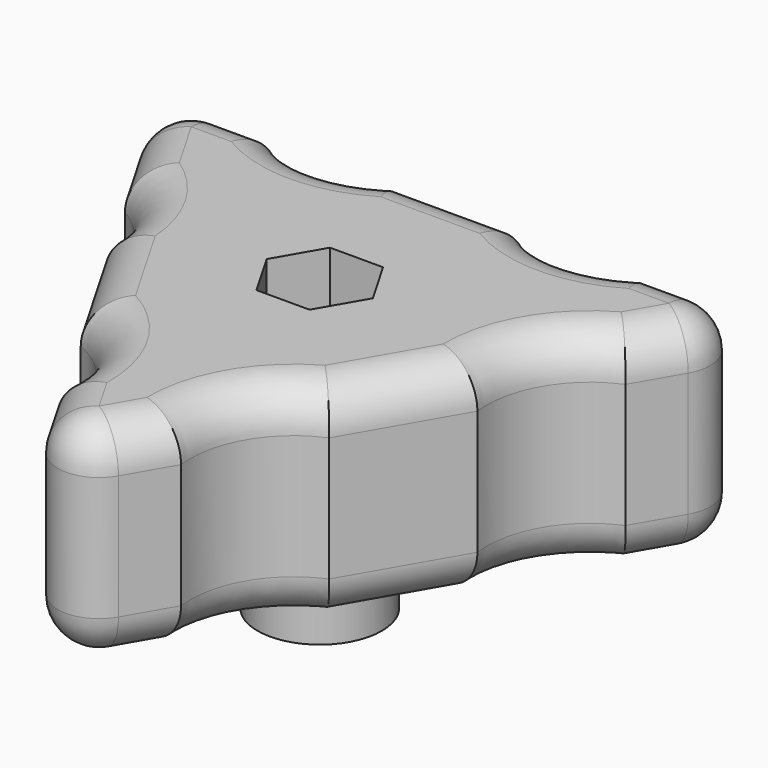
from build123d import *

# Parameters (mm, degrees)
F1_DEPTH     = 25.4
F2_R         = 5.08
F3_R         = 5.08
F4_T1_DEPTH  = 15.24
F4_T6_DEPTH  = 5.08
F4_T12_DEPTH = 5.08
F4_T18_DEPTH = 5.08
F4_T24_DEPTH = 5.08
F4_T30_DEPTH = 5.08
F4_T36_DEPTH = 5.08
F5_R         = 7.62
F6_DEPTH     = 10.16
F8_DEPTH     = 38.1


# Not quite as in the source:
# - a fillet or chamfer that OpenCascade refuses, or shapes differently, is made with other operations: its cross-section is extruded or revolved along the edge and cut away or added


with BuildPart() as f1:
    # F0 (on Top) → F1 (new body)
    with BuildSketch(Plane.XY):
        with BuildLine():
            Line((-22.8599986406, 21.9970466689), (-38.0999986406, 21.9970476107))
            Line((-38.0999986406, 21.9970476107), (-29.3011817939, 6.7570476107))
            ThreePointArc((-29.3011817939, 6.7570476107), (-24.5610386949, 2.0561338123), (-22.8600002719, -4.3994076385))
            Line((-22.8600002719, -4.3994076385), (-15.2400010875, -17.5976352631))
            ThreePointArc((-15.2400010875, -17.5976352631), (-9.2302968913, -22.9267492113), (-7.6200019032, -30.7958628877))
            Line((-7.6200019032, -30.7958628877), (-2.7189e-06, -43.9940905122))
            Line((-2.7189e-06, -43.9940905122), (7.6199980968, -30.7958638295))
            ThreePointArc((7.6199980968, -30.7958638295), (9.2302940575, -22.9267503522), (15.2399989124, -17.5976371467))
            Line((15.2399989124, -17.5976371467), (22.8599997281, -4.399410464))
            ThreePointArc((22.8599997281, -4.399410464), (24.4702956888, 3.4697030133), (30.4800005438, 8.7988162188))
            Line((30.4800005438, 8.7988162188), (38.1000013594, 21.9970429015))
            Line((38.1000013594, 21.9970429015), (22.8600013594, 21.9970438434))
            ThreePointArc((22.8600013594, 21.9970438434), (15.2400012025, 19.4570443143), (7.6200013594, 21.9970447852))
            Line((7.6200013594, 21.9970447852), (-7.6199986406, 21.997045727))
            ThreePointArc((-7.6199986406, 21.997045727), (-15.2399987975, 19.457046198), (-22.8599986406, 21.9970466689))
        make_face()
    extrude(amount=F1_DEPTH)

    # F2
    f2_edges = [f1.edges().sort_by_distance(p)[0] for p in [
        (-30.479999, 21.997047, 25.4),
        (-33.70059, 14.377048, 25.4),
        (-24.561039, 2.056134, 25.4),
        (-19.050001, -10.998521, 25.4),
        (-9.230297, -22.926749, 25.4),
        (-3.810002, -37.394977, 25.4),
        (3.809998, -37.394977, 25.4),
        (9.230294, -22.92675, 25.4),
        (19.049999, -10.998524, 25.4),
        (24.470296, 3.469703, 25.4),
        (34.290001, 15.39793, 25.4),
        (30.480001, 21.997043, 25.4),
        (15.240001, 19.457044, 25.4),
        (1e-06, 21.997045, 25.4),
        (-15.239999, 19.457046, 25.4),
    ]]
    fillet(f2_edges, radius=F2_R)

    # F3
    f3_edges = [f1.edges().sort_by_distance(p)[0] for p in [
        (-30.479999, 21.997047, 0),
        (-33.70059, 14.377048, 0),
        (-24.561039, 2.056134, 0),
        (-19.050001, -10.998521, 0),
        (-9.230297, -22.926749, 0),
        (-3.810002, -37.394977, 0),
        (3.809998, -37.394977, 0),
        (9.230294, -22.92675, 0),
        (19.049999, -10.998524, 0),
        (24.470296, 3.469703, 0),
        (34.290001, 15.39793, 0),
        (30.480001, 21.997043, 0),
        (15.240001, 19.457044, 0),
        (1e-06, 21.997045, 0),
        (-15.239999, 19.457046, 0),
    ]]
    fillet(f3_edges, radius=F3_R)

    # F4: fillet of radius 5.08 on 3 edges, made by hand

    # F4_s2 → F4_t1 (cut)
    with BuildSketch(Plane.XY.offset(5.08)):
        with BuildLine():
            ThreePointArc((-4.3994112992, -36.3740902404), (-2.4049e-06, -38.9140905122), (4.3994068033, -36.3740907841))
            Line((4.3994068033, -36.3740907841), (-2.7189e-06, -43.9940905122))
            Line((-2.7189e-06, -43.9940905122), (-4.3994112992, -36.3740902404))
        make_face()
        with BuildLine():
            ThreePointArc((29.301183257, 21.9970434453), (33.7005921512, 19.4570431734), (33.7005918373, 14.3770431734))
            Line((33.7005918373, 14.3770431734), (38.1000013594, 21.9970429015))
            Line((38.1000013594, 21.9970429015), (29.301183257, 21.9970434453))
        make_face()
        with BuildLine():
            ThreePointArc((-29.3011805381, 21.997047067), (-33.7005897463, 19.4570473389), (-33.7005900603, 14.3770473389))
            Line((-33.7005900603, 14.3770473389), (-38.0999986406, 21.9970476107))
            Line((-38.0999986406, 21.9970476107), (-29.3011805381, 21.997047067))
        make_face()
    extrude(amount=F4_T1_DEPTH, mode=Mode.SUBTRACT)


with BuildPart() as f4_tool4:
    # F4_s5 → F4_t6 (new body)
    with BuildSketch(Plane.XY.offset(20.32)):
        Polygon((-29.3011808521, 16.917047067), (-29.3011805381, 21.997047067), (-38.0999986406, 21.9970476107), (-33.7005900603, 14.3770473389), align=None)
    extrude(amount=F4_T6_DEPTH)

    # F4_s7 → F4_t8 (revolve, cut)
    with BuildSketch(Plane(origin=(-29.3011808521, 16.917047067, 20.32), x_dir=(0.8660253729, -0.5000000535, 0), z_dir=(-0.5000000535, -0.8660253729, 0))):
        with BuildLine():
            ThreePointArc((0, -5.08), (5.08, 0), (0, 5.08))
            Line((0, 5.08), (0, -5.08))
        make_face()
    revolve(axis=Axis((-29.3011808521, 16.917047067, 20.32), (0, 0, 1)), mode=Mode.SUBTRACT)


with BuildPart() as f1_1:
    add(f1.part)

    # F4_t3: cut F4_tool4
    add(f4_tool4.part, mode=Mode.SUBTRACT)


with BuildPart() as f4_tool10:
    # F4_s11 → F4_t12 (new body)
    with BuildSketch(Plane.XY.offset(20.32)):
        Polygon((29.301182943, 16.9170434453), (29.301183257, 21.9970434453), (38.1000013594, 21.9970429015), (33.7005918373, 14.3770431734), align=None)
    extrude(amount=F4_T12_DEPTH)

    # F4_s13 → F4_t14 (revolve, cut)
    with BuildSketch(Plane(origin=(29.301182943, 16.9170434453, 20.32), x_dir=(-0.8660254347, -0.4999999465, 0), z_dir=(-0.4999999465, 0.8660254347, 0))):
        with BuildLine():
            ThreePointArc((0, -5.08), (5.08, 0), (0, 5.08))
            Line((0, 5.08), (0, -5.08))
        make_face()
    revolve(axis=Axis((29.301182943, 16.9170434453, 20.32), (0, 0, 1)), mode=Mode.SUBTRACT)


with BuildPart() as f1_2:
    add(f1_1.part)

    # F4_t9: cut F4_tool10
    add(f4_tool10.part, mode=Mode.SUBTRACT)


with BuildPart() as f4_tool16:
    # F4_s17 → F4_t18 (new body)
    with BuildSketch(Plane.XY.offset(5.08)):
        Polygon((-2.091e-06, -33.8340905122), (-4.3994112992, -36.3740902404), (-2.7189e-06, -43.9940905122), (4.3994068033, -36.3740907841), align=None)
    extrude(amount=-F4_T18_DEPTH)

    # F4_s19 → F4_t20 (revolve, cut)
    with BuildSketch(Plane(origin=(-2.091e-06, -33.8340905122, 5.08), x_dir=(6.18e-08, 1, 0), z_dir=(-1, 6.18e-08, 0))):
        with BuildLine():
            ThreePointArc((0, -5.08), (5.08, 0), (0, 5.08))
            Line((0, 5.08), (0, -5.08))
        make_face()
    revolve(axis=Axis((-2.091e-06, -33.8340905122, 5.08), (0, 0, -1)), mode=Mode.SUBTRACT)


with BuildPart() as f1_3:
    add(f1_2.part)

    # F4_t15: cut F4_tool16
    add(f4_tool16.part, mode=Mode.SUBTRACT)


with BuildPart() as f4_tool22:
    # F4_s23 → F4_t24 (new body)
    with BuildSketch(Plane.XY.offset(20.32)):
        Polygon((-2.091e-06, -33.8340905122), (-4.3994112992, -36.3740902404), (-2.7189e-06, -43.9940905122), (4.3994068033, -36.3740907841), align=None)
    extrude(amount=F4_T24_DEPTH)

    # F4_s25 → F4_t26 (revolve, cut)
    with BuildSketch(Plane(origin=(-2.091e-06, -33.8340905122, 20.32), x_dir=(6.18e-08, 1, 0), z_dir=(1, -6.18e-08, 0))):
        with BuildLine():
            ThreePointArc((0, -5.08), (5.08, 0), (0, 5.08))
            Line((0, 5.08), (0, -5.08))
        make_face()
    revolve(axis=Axis((-2.091e-06, -33.8340905122, 20.32), (0, 0, 1)), mode=Mode.SUBTRACT)


with BuildPart() as f1_4:
    add(f1_3.part)

    # F4_t21: cut F4_tool22
    add(f4_tool22.part, mode=Mode.SUBTRACT)


with BuildPart() as f4_tool28:
    # F4_s29 → F4_t30 (new body)
    with BuildSketch(Plane.XY.offset(5.08)):
        Polygon((29.301182943, 16.9170434453), (29.301183257, 21.9970434453), (38.1000013594, 21.9970429015), (33.7005918373, 14.3770431734), align=None)
    extrude(amount=-F4_T30_DEPTH)

    # F4_s31 → F4_t32 (revolve, cut)
    with BuildSketch(Plane(origin=(29.301182943, 16.9170434453, 5.08), x_dir=(-0.8660254347, -0.4999999465, 0), z_dir=(0.4999999465, -0.8660254347, 0))):
        with BuildLine():
            ThreePointArc((0, -5.08), (5.08, 0), (0, 5.08))
            Line((0, 5.08), (0, -5.08))
        make_face()
    revolve(axis=Axis((29.301182943, 16.9170434453, 5.08), (0, 0, -1)), mode=Mode.SUBTRACT)


with BuildPart() as f1_5:
    add(f1_4.part)

    # F4_t27: cut F4_tool28
    add(f4_tool28.part, mode=Mode.SUBTRACT)


with BuildPart() as f4_tool34:
    # F4_s35 → F4_t36 (new body)
    with BuildSketch(Plane.XY.offset(5.08)):
        Polygon((-29.3011808521, 16.917047067), (-29.3011805381, 21.997047067), (-38.0999986406, 21.9970476107), (-33.7005900603, 14.3770473389), align=None)
    extrude(amount=-F4_T36_DEPTH)

    # F4_s37 → F4_t38 (revolve, cut)
    with BuildSketch(Plane(origin=(-29.3011808521, 16.917047067, 5.08), x_dir=(0.8660253729, -0.5000000535, 0), z_dir=(0.5000000535, 0.8660253729, 0))):
        with BuildLine():
            ThreePointArc((0, -5.08), (5.08, 0), (0, 5.08))
            Line((0, 5.08), (0, -5.08))
        make_face()
    revolve(axis=Axis((-29.3011808521, 16.917047067, 5.08), (0, 0, -1)), mode=Mode.SUBTRACT)


with BuildPart() as f1_6:
    add(f1_5.part)

    # F4_t33: cut F4_tool34
    add(f4_tool34.part, mode=Mode.SUBTRACT)

    # F5 (on face) → F6 (join)
    with BuildSketch(Plane(origin=(0, 0, 0), x_dir=(1, 0, 0), z_dir=(0, 0, -1))):
        Circle(F5_R)
    extrude(amount=F6_DEPTH)

    # F7 (on face) → F8 (cut)
    with BuildSketch(Plane(origin=(0, 0, -10.16), x_dir=(1, 0, 0), z_dir=(0, 0, -1))):
        Polygon((-3.2555626979, -5.6388), (3.2555626979, -5.6388), (6.5111253958, 0), (3.2555626979, 5.6388), (-3.2555626979, 5.6388), (-6.5111253958, 0), align=None)
    extrude(amount=-F8_DEPTH, mode=Mode.SUBTRACT)


solid = f1_6.part
